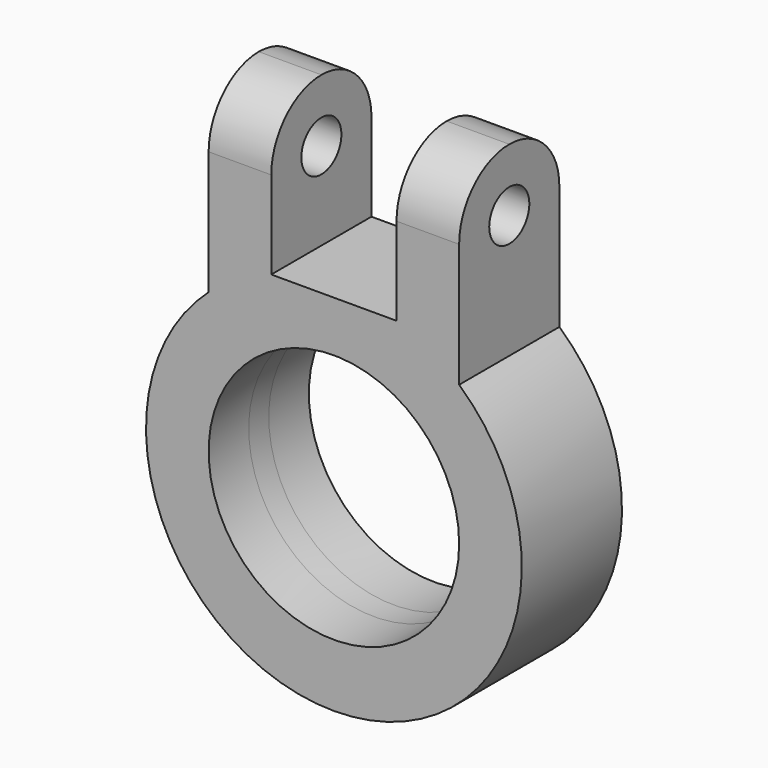
from build123d import *

# Parameters (mm, degrees)
F0_R          = 37.5
F0_R_2        = 25
F1_DEPTH      = 5
F2_W          = 5
F2_H          = 10
F3_DEPTH      = 5
F4_R          = 2.49999
F5_R          = 37.5
F5_R_2        = 25
F6_DEPTH      = 10
F6_DEPTH_BACK = 15
F7_W          = 50
F7_H          = 40
F8_DEPTH      = 15
F8_DEPTH_BACK = 10
F9_W          = 25
F9_H          = 30
F10_DEPTH     = 25
F11_R         = 12.49999
F12_R         = 5
F13_DEPTH     = 62.501


# Not quite as in the source:
# - a fillet or chamfer is up to 0.001 mm smaller than in the source, because OpenCascade refuses the exact size


with BuildPart() as f1:
    # F0 (on Front) → F1 (new body)
    with BuildSketch(Plane.XZ):
        Circle(F0_R)
        Circle(F0_R_2, mode=Mode.SUBTRACT)
    extrude(amount=F1_DEPTH)

    # F2 (on Front) → F3 (join)
    with BuildSketch(Plane.XZ):
        with Locations((0, 25)):
            Rectangle(F2_W, F2_H)
    extrude(amount=F3_DEPTH)

    # F4 (radius 2.5 in the source; OpenCascade refuses exactly that, so slightly less here)
    f4_edges = [f1.edges().sort_by_distance(p)[0] for p in [
        (-2.5, -5, 22.437343),
        (2.5, -5, 22.437343),
        (-2.5, 0, 22.437343),
        (2.5, 0, 22.437343),
    ]]
    fillet(f4_edges, radius=F4_R)

    # F5 (on face) → F6 (join, two sides)
    with BuildSketch(Plane.XZ.offset(5)) as f6_sk:
        Circle(F5_R)
        Circle(F5_R_2, mode=Mode.SUBTRACT)
    extrude(amount=F6_DEPTH)
    extrude(f6_sk.sketch, amount=-F6_DEPTH_BACK)

    # F7 (on Front) → F8 (join, two sides)
    with BuildSketch(Plane.XZ) as f8_sk:
        with Locations((0, 45.1250001788)):
            Rectangle(F7_W, F7_H)
    extrude(amount=F8_DEPTH)
    extrude(f8_sk.sketch, amount=-F8_DEPTH_BACK)

    # F9 (on face) → F10 (cut)
    with BuildSketch(Plane.XZ.offset(15)):
        with Locations((0, 50.1250001788)):
            Rectangle(F9_W, F9_H)
    extrude(amount=-F10_DEPTH, mode=Mode.SUBTRACT)

    # F11 (radius 12.5 in the source; OpenCascade refuses exactly that, so slightly less here)
    f11_edges = [f1.edges().sort_by_distance(p)[0] for p in [
        (-18.75, 10, 65.125),
        (-18.75, -15, 65.125),
        (18.75, -15, 65.125),
        (18.75, 10, 65.125),
    ]]
    fillet(f11_edges, radius=F11_R)

    # F12 (on face) → F13 (cut, through all)
    with BuildSketch(Plane(origin=(-25, 0, 0), x_dir=(0, -1, 0), z_dir=(-1, 0, 0))):
        with Locations((2.5, 52.6250001788)):
            Circle(F12_R)
    extrude(amount=-F13_DEPTH, mode=Mode.SUBTRACT)


solid = f1.part
